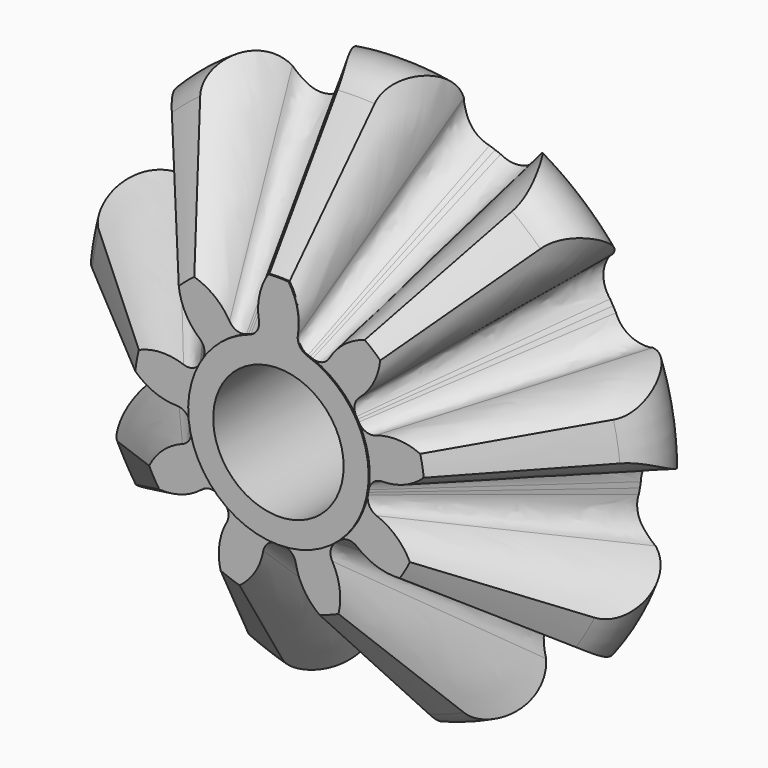
from build123d import *

# Parameters (mm, degrees)
F2_R             = 6.59
F3_DEPTH         = 0.05
F5_DEPTH         = 0.05
F7_DEPTH         = 0.05
F24_COPIES_COUNT = 9
F25_R            = 3.175
F26_R            = 4.7625
F27_DEPTH        = 12.7510001


# Not quite as in the source:
# - a pattern or mirror of a feature is missing from the dataset's text; its kind, count and spacing are read off the source's solid


with BuildPart() as f3:
    # F2 (on Front) → F3 (new body, symmetric)
    with BuildSketch(Plane.XZ):
        Circle(F2_R)
    extrude(amount=F3_DEPTH, both=True)

    # F4 (on Front) → F5 (join, symmetric)
    with BuildSketch(Plane.XZ):
        with BuildLine():
            ThreePointArc((-1.1776872799, 6.4839149185), (0, 6.59), (1.1776872799, 6.4839149185))
            ThreePointArc((1.1776872799, 6.4839149185), (1.4579597768, 8.5777511061), (0.7390671926, 10.5641790824))
            ThreePointArc((0.7390671926, 10.5641790824), (0, 10.59), (-0.7390671926, 10.5641790824))
            ThreePointArc((-0.7390671926, 10.5641790824), (-1.4579597768, 8.5777511061), (-1.1776872799, 6.4839149185))
        make_face()
    extrude(amount=F5_DEPTH, both=True)

    # F6 (on Front) → F7 (join, symmetric)
    with BuildSketch(Plane.XZ):
        with BuildLine():
            ThreePointArc((2.0903855568, 6.2496710492), (1.5501113208, 6.6835104035), (1.4215242077, 7.3643761684))
            Line((1.4215242077, 7.3643761684), (-1.4215242077, 7.3643761684))
            ThreePointArc((-1.4215242077, 7.3643761684), (-1.5501113208, 6.6835104035), (-2.0903855568, 6.2496710492))
            ThreePointArc((-2.0903855568, 6.2496710492), (0, 6.59), (2.0903855568, 6.2496710492))
        make_face()
    extrude(amount=F7_DEPTH, both=True)

    # F23 (on face) → F24 section 0
    with BuildSketch(Plane(origin=(0, 0.05, 0), x_dir=(-1, 0, 0), z_dir=(0, 1, 0))):
        with BuildLine():
            ThreePointArc((-0.7390671926, 10.5641790824), (-1.3857142859, 9.0294175925), (-1.4215242077, 7.3643761684))
            ThreePointArc((-1.4215242077, 7.3643761684), (-1.5501113208, 6.6835104035), (-2.0903855568, 6.2496710492))
            ThreePointArc((-2.0903855568, 6.2496710492), (-2.1723367466, 6.2216599923), (-2.2539127445, 6.192574371))
            Line((-2.2539127445, 6.192574371), (0, 0))
            Line((0, 0), (2.2539127445, 6.192574371))
            ThreePointArc((2.2539127445, 6.192574371), (2.1723367466, 6.2216599923), (2.0903855568, 6.2496710492))
            ThreePointArc((2.0903855568, 6.2496710492), (1.5501113208, 6.6835104035), (1.4215242077, 7.3643761684))
            ThreePointArc((1.4215242077, 7.3643761684), (1.3857142859, 9.0294175925), (0.7390671926, 10.5641790824))
            ThreePointArc((0.7390671926, 10.5641790824), (0, 10.59), (-0.7390671926, 10.5641790824))
        make_face()
    # F22 (on offset) → F24 section 1
    with BuildSketch(Plane.XZ.offset(-12.7)):
        with BuildLine():
            ThreePointArc((3.5503431795, 18.3929774522), (3.2488716636, 22.5206123027), (1.8479820326, 26.4149367339))
            ThreePointArc((1.8479820326, 26.4149367339), (0, 26.4795), (-1.8479820326, 26.4149367339))
            ThreePointArc((-1.8479820326, 26.4149367339), (-3.2488716636, 22.5206123027), (-3.5503431795, 18.3929774522))
            ThreePointArc((-3.5503431795, 18.3929774522), (-3.7544889645, 16.620033345), (-5.2169235296, 15.5971494555))
            ThreePointArc((-5.2169235296, 15.5971494555), (-5.4214470868, 15.5272429534), (-5.6250342872, 15.4546546878))
            Line((-5.6250342872, 15.4546546878), (0, 0))
            Line((0, 0), (5.6250342872, 15.4546546878))
            ThreePointArc((5.6250342872, 15.4546546878), (5.4214470868, 15.5272429534), (5.2169235296, 15.5971494555))
            ThreePointArc((5.2169235296, 15.5971494555), (3.7544889645, 16.620033345), (3.5503431795, 18.3929774522))
        make_face()
    f24 = loft()

    # F24_copies: F24 ×9 about axis
    f24_copies_axis = Axis((0, 0, 0), (0, 1, 0))
    for i in range(1, F24_COPIES_COUNT):
        add(f24.rotate(f24_copies_axis, i * 360 / F24_COPIES_COUNT))

    # F25
    f25_edges = [f3.edges().sort_by_distance(p)[0] for p in [
        (0, 12.7, 26.4795),
        (-26.077217, 12.7, 4.598117),
        (-22.93192, 12.7, -13.23975),
        (-9.056522, 12.7, -24.882591),
        (9.056522, 12.7, -24.882591),
        (22.93192, 12.7, -13.23975),
        (26.077217, 12.7, 4.598117),
        (17.020695, 12.7, 20.284474),
        (-17.020695, 12.7, 20.284474),
    ]]
    fillet(f25_edges, radius=F25_R)

    # F26 (on face) → F27 (cut, through all)
    with BuildSketch(Plane.XZ.offset(0.05)):
        Circle(F26_R)
    extrude(amount=-F27_DEPTH, mode=Mode.SUBTRACT)


solid = f3.part
